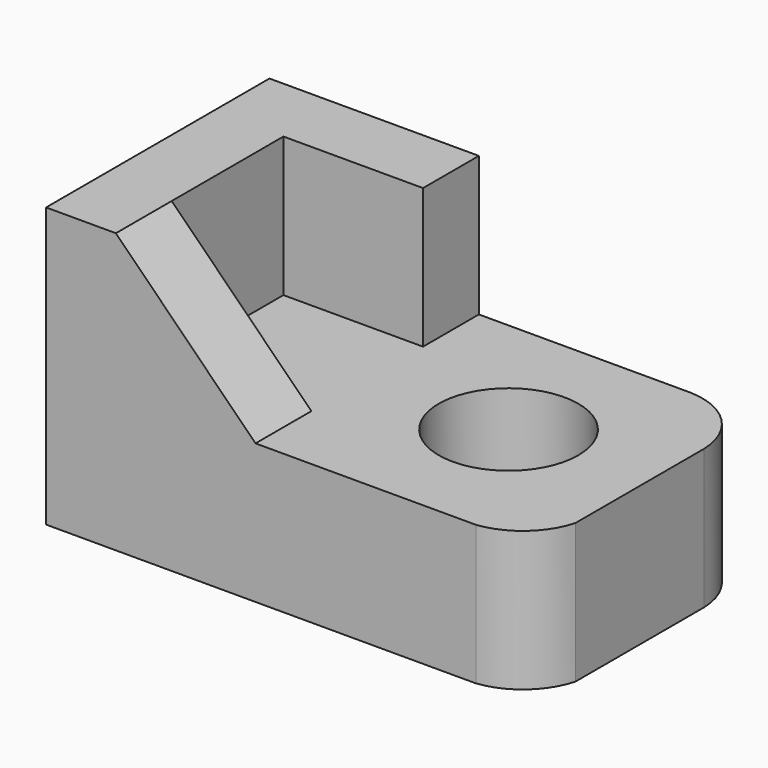
from build123d import *

# Parameters (mm, degrees)
F1_DEPTH  = 40
F3_DEPTH  = 10
F4_W      = 20
F4_H      = 20
F5_DEPTH  = 20
F7_DEPTH  = 20
F9_DEPTH  = 20
F11_DEPTH = 20


with BuildPart() as f1:
    # F0 (on Front) → F1 (new body)
    with BuildSketch(Plane.XZ):
        Polygon((0, 40), (0, 0), (70, 0), (70, 20), (30, 20), (30, 40), align=None)
    extrude(amount=F1_DEPTH)

    # F2 (on face) → F3 (cut)
    with BuildSketch(Plane.XZ.offset(40)):
        Polygon((30, 20), (30, 40), (10, 40), align=None)
    extrude(amount=-F3_DEPTH, mode=Mode.SUBTRACT)

    # F4 (on face) → F5 (cut)
    with BuildSketch(Plane.XY.offset(40)):
        with Locations((20, -20)):
            Rectangle(F4_W, F4_H)
    extrude(amount=-F5_DEPTH, mode=Mode.SUBTRACT)

    # F6 (on face) → F7 (cut)
    with BuildSketch(Plane.XY.offset(20)):
        with BuildLine():
            ThreePointArc((60.3829629344, 0), (67.0878115757, -2.9325770906), (70, -9.6463064772))
            Line((70, -9.6463064772), (70, 0))
            Line((70, 0), (60.3829629344, 0))
        make_face()
    extrude(amount=-F7_DEPTH, mode=Mode.SUBTRACT)

    # F8 (on face) → F9 (cut)
    with BuildSketch(Plane.XY.offset(20)):
        with BuildLine():
            ThreePointArc((70, -32.718077302), (66.9100377104, -37.6307978482), (61.6119652987, -40))
            Line((61.6119652987, -40), (70, -40))
            Line((70, -40), (70, -32.718077302))
        make_face()
    extrude(amount=-F9_DEPTH, mode=Mode.SUBTRACT)

    # F10 (on face) → F11 (cut)
    with BuildSketch(Plane.XY.offset(20)):
        with BuildLine():
            ThreePointArc((50, -29.687499851), (57.0710678119, -26.7585676629), (60, -19.687499851))
            ThreePointArc((60, -19.687499851), (42.9289321881, -12.6164320391), (50, -29.687499851))
        make_face()
    extrude(amount=-F11_DEPTH, mode=Mode.SUBTRACT)


solid = f1.part
